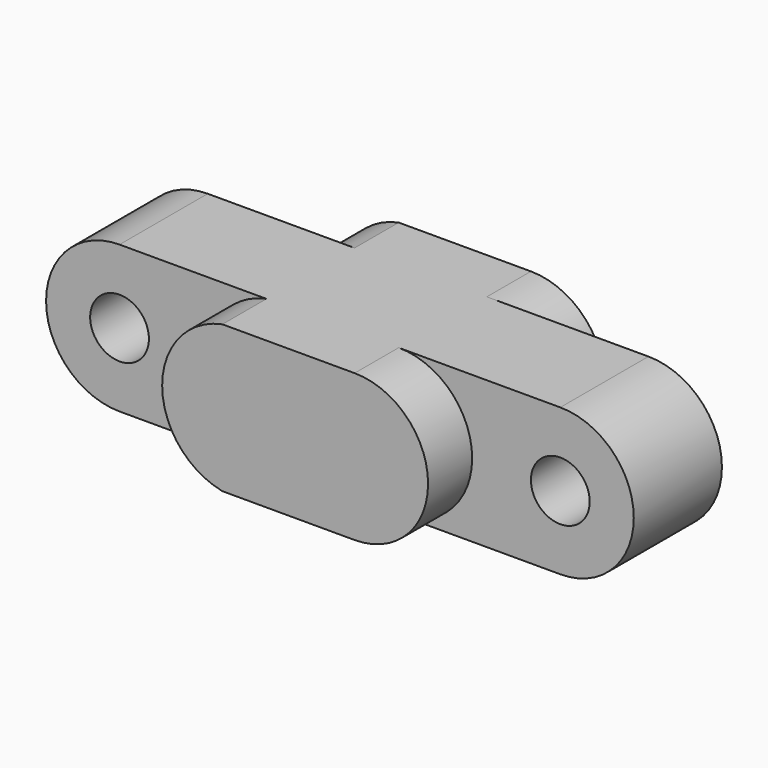
from build123d import *

# Parameters (mm, degrees)
F0_R          = 0.4
F1_DEPTH      = 1.5
F2_DEPTH      = 0.75
F2_DEPTH_BACK = 2.25


# Not quite as in the source:
# - a feature names something its author has since deleted; it is built from what else it names


with BuildPart() as f1:
    # F0 (on Front) → F1 (new body)
    with BuildSketch(Plane.XZ):
        with BuildLine():
            ThreePointArc((-2.2, -2.24940907), (-1.2, -1.24940907), (-2.2, -0.24940907))
            Line((-2.2, -0.24940907), (-4, -0.24940907))
            ThreePointArc((-4, -0.24940907), (-4.8198039027, -1.24940907), (-4, -2.24940907))
            Line((-4, -2.24940907), (-2.2, -2.24940907))
        make_face()
        with BuildLine():
            Line((0, -0.24940907), (-1, -0.24940907))
            Line((-1, -0.24940907), (-2.2, -0.24940907))
            ThreePointArc((-2.2, -0.24940907), (-1.2, -1.24940907), (-2.2, -2.24940907))
            Line((-2.2, -2.24940907), (-1, -2.24940907))
            Line((-1, -2.24940907), (0, -2.24940907))
            ThreePointArc((0, -2.24940907), (1, -1.24940907), (0, -0.24940907))
        make_face()
        with Locations((0, -1.24940907)):
            Circle(F0_R, mode=Mode.SUBTRACT)
        with BuildLine():
            ThreePointArc((-4, -2.24940907), (-4.8198039027, -1.24940907), (-4, -0.24940907))
            Line((-4, -0.24940907), (-6, -0.24940907))
            ThreePointArc((-6, -0.24940907), (-7, -1.24940907), (-6, -2.24940907))
            Line((-6, -2.24940907), (-4, -2.24940907))
        make_face()
        with Locations((-6, -1.24940907)):
            Circle(F0_R, mode=Mode.SUBTRACT)
    extrude(amount=F1_DEPTH)

    # F0 (on Front) → F2 (join, two sides)
    with BuildSketch(Plane.XZ) as f2_sk:
        with BuildLine():
            ThreePointArc((-2.2, -2.24940907), (-1.2, -1.24940907), (-2.2, -0.24940907))
            Line((-2.2, -0.24940907), (-4, -0.24940907))
            ThreePointArc((-4, -0.24940907), (-4.8198039027, -1.24940907), (-4, -2.24940907))
            Line((-4, -2.24940907), (-2.2, -2.24940907))
        make_face()
    extrude(amount=-F2_DEPTH)
    extrude(f2_sk.sketch, amount=F2_DEPTH_BACK)


solid = f1.part
